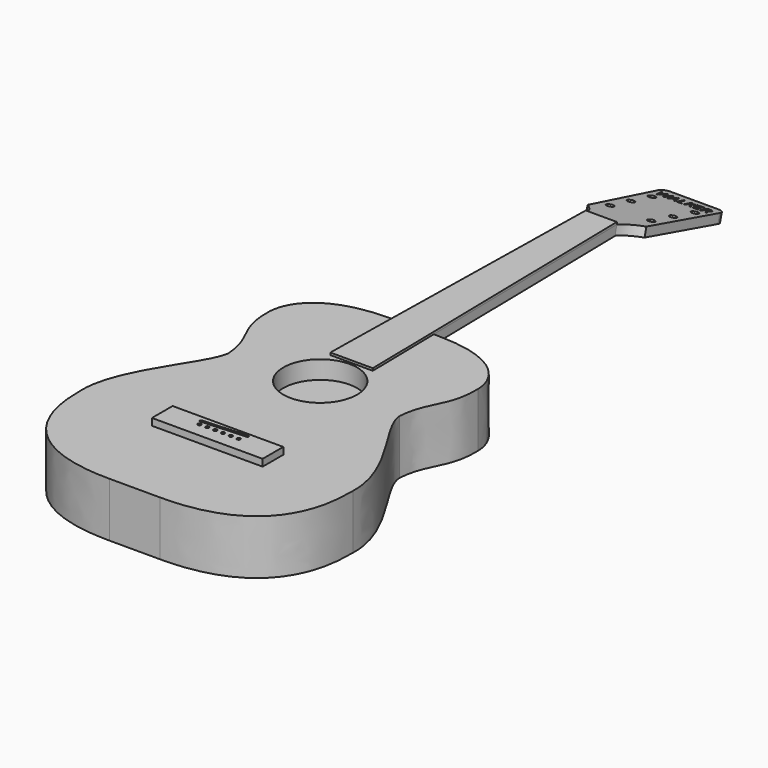
from build123d import *

# Parameters (mm, degrees)
F5_R         = 4.7625
F7_DEPTH     = 12.5
F6_TEXT_SIZE = 19.0261946524
F8_DEPTH     = 3.175
F9_DEPTH     = 3.175
F10_DEPTH    = 12.5
F11_DEPTH    = 75
F1_R         = 50.8
F12_DEPTH    = 25
F2_R         = 2.38125
F13_DEPTH    = 9.525


# Not quite as in the source:
# - Text() gives the source's letters only with a copy of the font that has no kerning and outlines rounded to 1/6400 em; it was checked with that copy


with BuildPart() as f7:
    # F5 (on 3pt) → F7 (new body)
    with BuildSketch(Plane(origin=(0, 53.7961593644, 200.77), x_dir=(1, 0, 0), z_dir=(0, 0.2588190451, 0.9659258263))):
        with BuildLine():
            Line((32.6904736233, 941.7759180088), (0, 941.7759180088))
            Line((0, 941.7759180088), (-32.6904736233, 941.7759180088))
            Line((-32.6904736233, 941.7759180088), (-33.626069305, 941.7759180088))
            ThreePointArc((-33.626069305, 941.7759180088), (-39.8520121637, 938.9835868414), (-42.5445994902, 932.7138618621))
            Line((-42.5445994902, 932.7138618621), (-42.5295011788, 931.7759180088))
            Line((-42.5295011788, 931.7759180088), (-40.4685344599, 803.7436498648))
            ThreePointArc((-40.4685344599, 803.7436498648), (-28.6031202921, 791.3236681231), (-21.43125, 775.7157125762))
            Line((-21.43125, 775.7157125762), (21.43125, 775.7157125762))
            ThreePointArc((21.43125, 775.7157125762), (28.6031202921, 791.3236681231), (40.4685344599, 803.7436498648))
            Line((40.4685344599, 803.7436498648), (42.5295011788, 931.7759180088))
            Line((42.5295011788, 931.7759180088), (42.5445994902, 932.7138618621))
            ThreePointArc((42.5445994902, 932.7138618621), (39.8520121637, 938.9835868414), (33.626069305, 941.7759180088))
            Line((33.626069305, 941.7759180088), (32.6904736233, 941.7759180088))
        make_face()
        with Locations((-28.3590368927, 828.1032125762)):
            Circle(F5_R, mode=Mode.SUBTRACT)
        with Locations((28.3590368927, 828.1032125762)):
            Circle(F5_R, mode=Mode.SUBTRACT)
        with Locations((-28.9723419065, 866.2032125762)):
            Circle(F5_R, mode=Mode.SUBTRACT)
        with Locations((-29.5856469204, 904.3032125762)):
            Circle(F5_R, mode=Mode.SUBTRACT)
        with Locations((28.9723419065, 866.2032125762)):
            Circle(F5_R, mode=Mode.SUBTRACT)
        with Locations((29.5856469204, 904.3032125762)):
            Circle(F5_R, mode=Mode.SUBTRACT)
        with BuildLine():
            ThreePointArc((33.626069305, 941.7759180088), (33.1582714642, 941.7875756646), (32.6904736233, 941.7759180088))
            Line((32.6904736233, 941.7759180088), (33.626069305, 941.7759180088))
        make_face()
        with BuildLine():
            Line((-33.626069305, 941.7759180088), (-32.6904736233, 941.7759180088))
            ThreePointArc((-32.6904736233, 941.7759180088), (-33.1582714642, 941.7875756646), (-33.626069305, 941.7759180088))
        make_face()
        with BuildLine():
            ThreePointArc((42.5295011787, 931.7759180088), (42.5487681372, 932.2447013111), (42.5445994902, 932.7138618621))
            Line((42.5445994902, 932.7138618621), (42.5295011788, 931.7759180088))
        make_face()
        with BuildLine():
            Line((-42.5295011788, 931.7759180088), (-42.5445994902, 932.7138618621))
            ThreePointArc((-42.5445994902, 932.7138618621), (-42.5487681372, 932.2447013111), (-42.5295011787, 931.7759180088))
        make_face()
    extrude(amount=-F7_DEPTH)

    # F6 (on 3pt) → F8 (cut)
    with BuildSketch(Plane(origin=(0, 53.7961593644, 200.77), x_dir=(1, 0, 0), z_dir=(0, 0.2588190451, 0.9659258263))):
        with Locations((-37.2289118176, 917.2067642212)):
            Text('WALKER', F6_TEXT_SIZE, font='Open Sans', text_align=(TextAlign.LEFT, TextAlign.BOTTOM))
    extrude(amount=-F8_DEPTH, mode=Mode.SUBTRACT)


with BuildPart() as f9:
    # F1 (on Top) → F9 (new body)
    with BuildSketch(Plane.XY):
        Polygon((21.43125, 803.08), (0, 803.08), (-21.43125, 803.08), (-27.2996771202, 480.5632032898), (-22.5375965251, 480.5), (0, 480.5), (22.5375965251, 480.5), (27.2996771202, 480.5632032898), align=None)
        Polygon((29.2530392665, 373.2104), (27.2996771202, 480.5632032898), (22.5375965251, 480.5), (0, 480.5), (-22.5375965251, 480.5), (-27.2996771202, 480.5632032898), (-29.2530392665, 373.2104), (0, 373.2104), align=None)
    extrude(amount=F9_DEPTH)


with BuildPart() as f10:
    # F1 (on Top) → F10 (new body)
    with BuildSketch(Plane.XY):
        Polygon((21.43125, 803.08), (0, 803.08), (-21.43125, 803.08), (-27.2996771202, 480.5632032898), (-22.5375965251, 480.5), (0, 480.5), (22.5375965251, 480.5), (27.2996771202, 480.5632032898), align=None)
        Polygon((29.2530392665, 373.2104), (27.2996771202, 480.5632032898), (22.5375965251, 480.5), (0, 480.5), (-22.5375965251, 480.5), (-27.2996771202, 480.5632032898), (-29.2530392665, 373.2104), (0, 373.2104), align=None)
    extrude(amount=-F10_DEPTH)


with BuildPart() as f11:
    # F0 (on Top) → F11 (new body)
    with BuildSketch(Plane.XY):
        with BuildLine():
            add(Edge.make_bspline(
                [(35, 480.5), (114.4532263279, 480.0247550011), (143.2027938366, 442.6989555359), (144, 411)],
                knots=[0, 0, 0, 0, 129.2720000619, 129.2720000619, 129.2720000619, 129.2720000619], degree=3))
            Line((35, 480.5), (0, 480.5))
            Line((0, 480.5), (-35, 480.5))
            add(Edge.make_bspline(
                [(-35, 480.5), (-114.4532263279, 480.0247550011), (-143.2027938366, 442.6989555359), (-144, 411)],
                knots=[0, 0, 0, 0, 129.2720000619, 129.2720000619, 129.2720000619, 129.2720000619], degree=3))
            add(Edge.make_bspline(
                [(-144, 411), (-145.6498327255, 360.7651293278), (-120.3481480479, 352.5278568268), (-117.5, 309)],
                knots=[0, 0, 0, 0, 105.3861945418, 105.3861945418, 105.3861945418, 105.3861945418], degree=3))
            add(Edge.make_bspline(
                [(-117.5, 309), (-118.7006905675, 277.5685191154), (-189.6336376667, 207.8346908092), (-187.3, 141.2)],
                knots=[0, 0, 0, 0, 181.7384934459, 181.7384934459, 181.7384934459, 181.7384934459], degree=3))
            add(Edge.make_bspline(
                [(-187.3, 141.2), (-186.8100183249, 117.8550839186), (-191.9634789228, 0), (-35, 0)],
                knots=[0, 0, 0, 0, 207.6842073919, 207.6842073919, 207.6842073919, 207.6842073919], degree=3))
            Line((-35, 0), (0, 0))
            Line((0, 0), (35, 0))
            add(Edge.make_bspline(
                [(187.3, 141.2), (186.8100183249, 117.8550839186), (191.9634789228, 0), (35, 0)],
                knots=[0, 0, 0, 0, 207.6842073919, 207.6842073919, 207.6842073919, 207.6842073919], degree=3))
            add(Edge.make_bspline(
                [(117.5, 309), (118.7006905675, 277.5685191154), (189.6336376667, 207.8346908092), (187.3, 141.2)],
                knots=[0, 0, 0, 0, 181.7384934459, 181.7384934459, 181.7384934459, 181.7384934459], degree=3))
            add(Edge.make_bspline(
                [(144, 411), (145.6498327255, 360.7651293278), (120.3481480479, 352.5278568268), (117.5, 309)],
                knots=[0, 0, 0, 0, 105.3861945418, 105.3861945418, 105.3861945418, 105.3861945418], degree=3))
        make_face()
    extrude(amount=-F11_DEPTH)

    # F1 (on Top) → F12 (cut)
    with BuildSketch(Plane.XY):
        with Locations((0, 319.2354)):
            Circle(F1_R)
    extrude(amount=-F12_DEPTH, mode=Mode.SUBTRACT)


with BuildPart() as f13:
    # F2 (on Top) → F13 (new body)
    with BuildSketch(Plane.XY):
        Polygon((76.2, 160.4219), (0, 160.4219), (-76.2, 160.4219), (-76.2, 124.8619), (0, 124.8619), (76.2, 124.8619), align=None)
        with Locations((-26.9875, 145.22)):
            Circle(F2_R, mode=Mode.SUBTRACT)
        with Locations((-16.1923, 145.22)):
            Circle(F2_R, mode=Mode.SUBTRACT)
        with Locations((-5.3971, 145.22)):
            Circle(F2_R, mode=Mode.SUBTRACT)
        with BuildLine():
            Line((-30.8222501914, 153.8424121339), (-26.9847128124, 154.0691366224))
            Line((-26.9847128124, 154.0691366224), (26.7553187995, 157.2441366224))
            Line((26.7553187995, 157.2441366224), (30.5928561785, 157.4708611108))
            ThreePointArc((30.5928561785, 157.4708611108), (32.2712201885, 155.9797518762), (30.7801109539, 154.3013878661))
            Line((30.7801109539, 154.3013878661), (26.942573575, 154.0746633776))
            Line((26.942573575, 154.0746633776), (-26.797458037, 150.8996633776))
            Line((-26.797458037, 150.8996633776), (-30.6349954159, 150.6729388892))
            ThreePointArc((-30.6349954159, 150.6729388892), (-32.313359426, 152.1640481238), (-30.8222501914, 153.8424121339))
        make_face(mode=Mode.SUBTRACT)
        with Locations((5.3971, 145.22)):
            Circle(F2_R, mode=Mode.SUBTRACT)
        with Locations((16.1923, 145.22)):
            Circle(F2_R, mode=Mode.SUBTRACT)
        with Locations((26.9875, 145.22)):
            Circle(F2_R, mode=Mode.SUBTRACT)
    extrude(amount=F13_DEPTH)


solid = Compound([f7.part, f9.part, f10.part, f11.part, f13.part])
